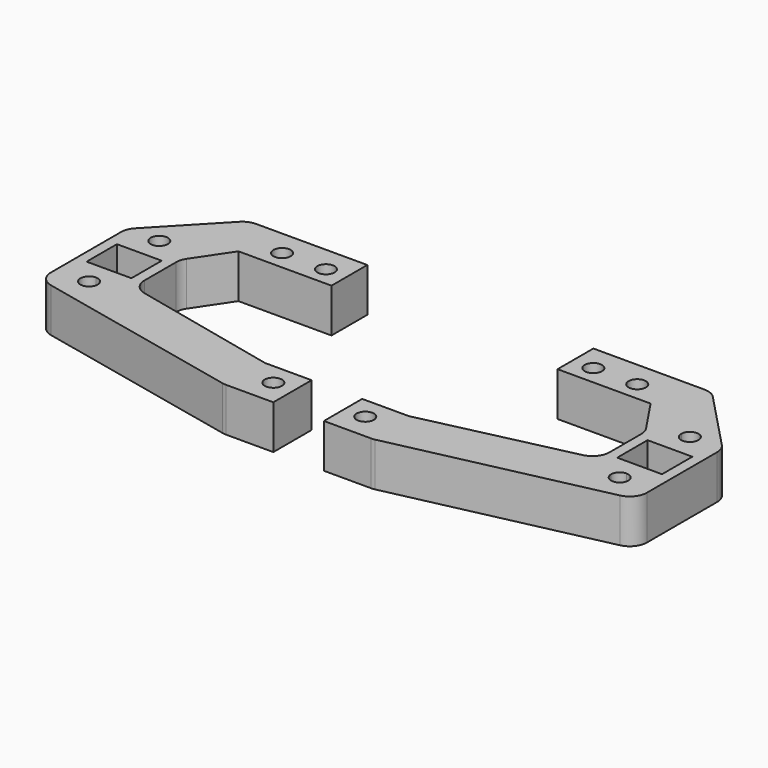
from build123d import *

# Parameters (mm, degrees)
F0_R     = 2.5
F1_DEPTH = 12.73
F0_R_2   = 1
F2_DEPTH = 3
F3_R     = 5
F4_R     = 5


# Not quite as in the source:
# - a feature names something its author has since deleted; it is built from what else it names


with BuildPart() as f1:
    # F0 (on Top) → F1 (new body)
    with BuildSketch(Plane.XY):
        Polygon((6, -5.5), (6, 5.5), (6, 7.5), (-28.4236618295, 7.5), (-47.69, -12.73), (-47.69, -16.96), (-38.19, -16.96), (-28.69, -16.96), (-21, -5.5), align=None)
        with BuildLine():
            ThreePointArc((-35.69, -12.73), (-36.422233047, -14.497766953), (-38.19, -15.23))
            ThreePointArc((-38.19, -15.23), (-39.957766953, -10.962233047), (-35.69, -12.73))
        make_face(mode=Mode.SUBTRACT)
        with Locations((-12.73, 0)):
            Circle(F0_R, mode=Mode.SUBTRACT)
        Circle(F0_R, mode=Mode.SUBTRACT)
        Polygon((17.9534775169, -44.5339671252), (-28.69, -33.96), (-38.19, -33.96), (-47.69, -33.96), (-47.69, -44.1913791001), (17.19, -58.42), (31.46, -58.42), (31.46, -44.5339671252), align=None)
        with BuildLine():
            ThreePointArc((-35.69, -38.19), (-39.957766953, -39.957766953), (-38.19, -35.69))
            ThreePointArc((-38.19, -35.69), (-36.422233047, -36.422233047), (-35.69, -38.19))
        make_face(mode=Mode.SUBTRACT)
        with Locations((25.46, -50.92)):
            Circle(F0_R, mode=Mode.SUBTRACT)
        Polygon((-28.69, -33.96), (-28.69, -16.96), (-38.19, -16.96), (-38.19, -19.96), (-31.69, -19.96), (-31.69, -30.96), (-38.19, -30.96), (-38.19, -33.96), align=None)
        Polygon((-38.19, -19.96), (-38.19, -16.96), (-47.69, -16.96), (-47.69, -33.96), (-38.19, -33.96), (-38.19, -30.96), (-44.69, -30.96), (-44.69, -19.96), align=None)
    extrude(amount=F1_DEPTH)

    # F0 (on Top) → F2 (join)
    with BuildSketch(Plane.XY):
        with BuildLine():
            Line((-38.19, -22.96), (-38.19, -19.96))
            Line((-38.19, -19.96), (-44.69, -19.96))
            Line((-44.69, -19.96), (-44.69, -30.96))
            Line((-44.69, -30.96), (-38.19, -30.96))
            Line((-38.19, -30.96), (-38.19, -27.96))
            ThreePointArc((-38.19, -27.96), (-40.69, -25.46), (-38.19, -22.96))
        make_face()
        with Locations((-42.69, -25.46)):
            Circle(F0_R_2, mode=Mode.SUBTRACT)
        with BuildLine():
            Line((-31.69, -19.96), (-38.19, -19.96))
            Line((-38.19, -19.96), (-38.19, -22.96))
            ThreePointArc((-38.19, -22.96), (-36.422233047, -23.692233047), (-35.69, -25.46))
            ThreePointArc((-35.69, -25.46), (-36.422233047, -27.227766953), (-38.19, -27.96))
            Line((-38.19, -27.96), (-38.19, -30.96))
            Line((-38.19, -30.96), (-31.69, -30.96))
            Line((-31.69, -30.96), (-31.69, -19.96))
        make_face()
        with Locations((-33.69, -25.46)):
            Circle(F0_R_2, mode=Mode.SUBTRACT)
    extrude(amount=F2_DEPTH)

    # F3
    f3_edges = [f1.edges().sort_by_distance(p)[0] for p in [
        (-28.423662, 7.5, 6.365),
        (-47.69, -12.73, 6.365),
        (-47.69, -44.191379, 6.365),
        (17.19, -58.42, 6.365),
    ]]
    fillet(f3_edges, radius=F3_R)

    # F4
    f4_edges = [f1.edges().sort_by_distance(p)[0] for p in [
        (-28.69, -16.96, 6.365),
        (-28.69, -33.96, 6.365),
    ]]
    fillet(f4_edges, radius=F4_R)


with BuildPart() as f1_1:
    # F5: moved
    add(f1.part.moved(Location((-38.8, 0, 0))))


with BuildPart() as f6_1:
    # F6: instance of F1
    add(f1_1.part.mirror(Plane.YZ))


solid = Compound([f1_1.part, f6_1.part])
